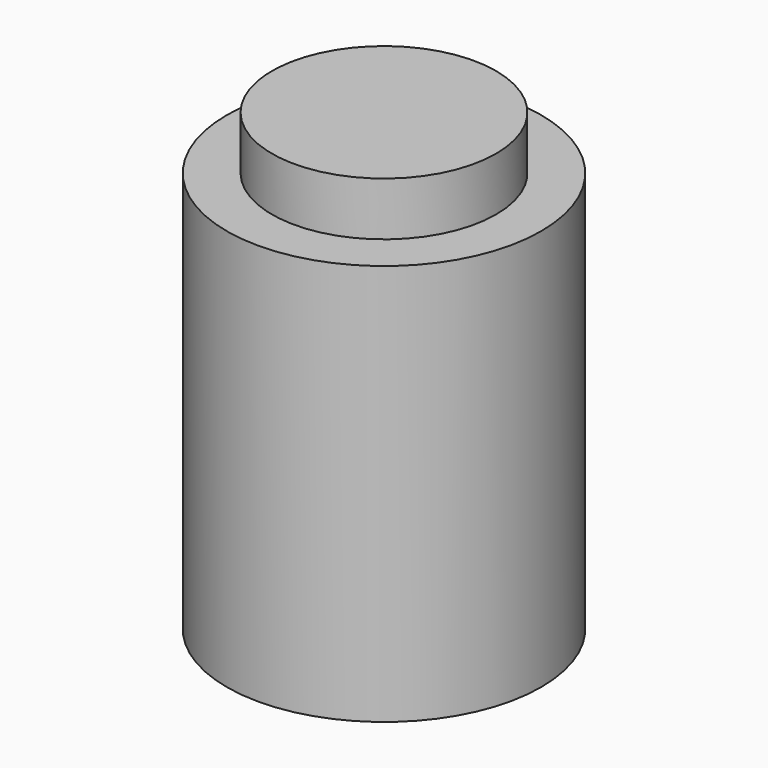
from build123d import *

# Parameters (mm, degrees)
F0_R     = 23.4960759557
F1_DEPTH = 60
F4_R     = 16.7480657564
F5_DEPTH = 8


# Not quite as in the source:
# - the program builds the solid bodies; features that only make, move or delete a surface that nothing else refers to are left out


with BuildPart() as f1:
    # F0 (on Top) → F1 (new body)
    with BuildSketch(Plane.XY):
        Circle(F0_R)
    extrude(amount=F1_DEPTH)

    # F4 (on face) → F5 (join)
    with BuildSketch(Plane.XY.offset(60)):
        Circle(F4_R)
    extrude(amount=F5_DEPTH)


solid = f1.part
